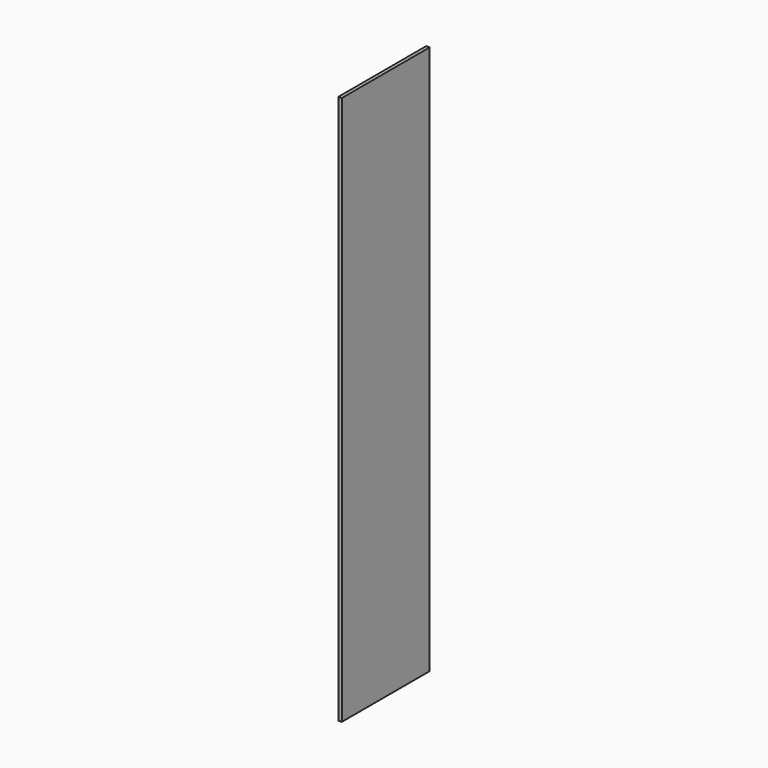
from build123d import *

# Parameters (mm, degrees)
F0_W     = 580
F0_H     = 2880
F1_DEPTH = 18


# Not quite as in the source:
# - a feature of the source that left no trace in its solid (it failed there, or was rolled back) is left out
# - a pattern or mirror of a feature is missing from the dataset's text; its kind, count and spacing are read off the source's solid


with BuildPart() as f1:
    # F0 (on Right) → F1 (new body)
    with BuildSketch(Plane.YZ):
        with Locations((290, 1440)):
            Rectangle(F0_W, F0_H)
    extrude(amount=F1_DEPTH)

    # F1_copies: F1 across plane


with BuildPart() as f1_1:
    add(f1.part)
    add(f1.part.mirror(Plane.XY.offset(1450)))


solid = f1_1.part
